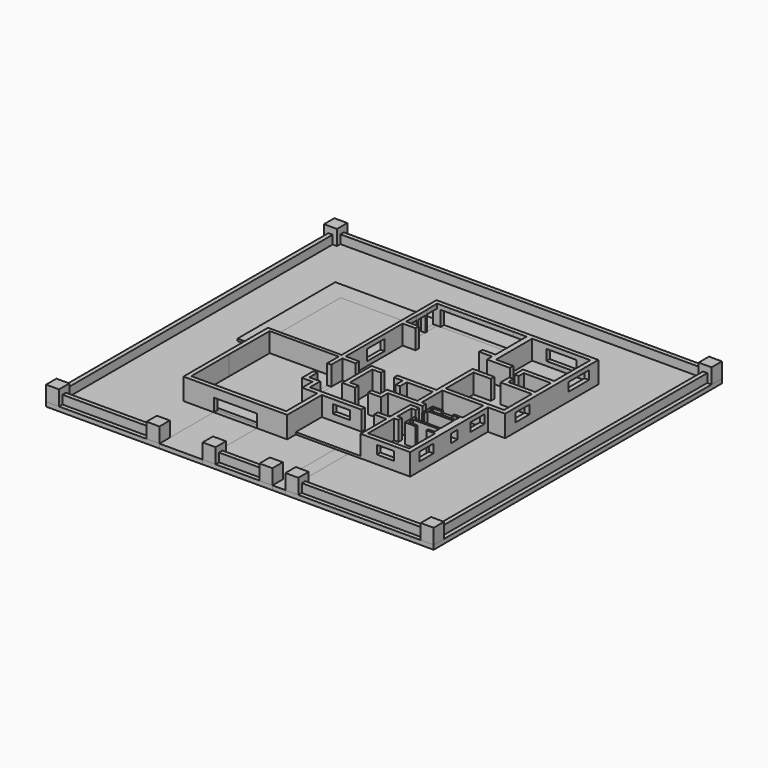
from build123d import *

# Parameters (mm, degrees)
F1_DEPTH  = 254
F2_DEPTH  = 254
F4_DEPTH  = 25.4
F5_W      = 203.2
F5_H      = 177.8
F6_DEPTH  = 50.8
F7_W      = 152.4
F7_H      = 254
F8_DEPTH  = 76.2
F9_W      = 939.5937236786
F9_H      = 25.4
F10_DEPTH = 53.34
F12_DEPTH = 63.5
F14_DEPTH = 76.2
F16_DEPTH = 101.6
F19_DEPTH = 76.2
F21_DEPTH = 76.2
F23_DEPTH = 76.2
F24_W     = 457.2
F24_H     = 177.8
F25_DEPTH = 76.2
F27_DEPTH = 76.2
F28_W     = 25.4
F28_H     = 25.4
F28_H_2   = 50.8
F28_H_3   = 177.8
F29_DEPTH = 50.8
F30_W     = 4055.1800727844
F30_H     = 3734.5069646835
F31_DEPTH = 50.8
F33_W     = 762
F33_H     = 1016
F34_DEPTH = 76.2
F35_W     = 762
F35_H     = 1016
F36_DEPTH = 76.2
F37_W     = 762
F37_H     = 1016
F38_DEPTH = 50.8
F39_DEPTH = 25.4
F40_DEPTH = 508
F41_DEPTH = 254
F42_DEPTH = 254
F44_W     = 3.137548542
F44_H     = 25.4
F44_W_2   = 758.862451458
F45_DEPTH = 381
F46_W     = 152.4
F46_H     = 50.8
F47_DEPTH = 1016
F48_DEPTH = 1016
F49_W     = 152.4
F49_H     = 152.4
F50_DEPTH = 177.8
F52_DEPTH = 1524
F53_W     = 152.4
F53_H     = 152.4
F54_DEPTH = 177.8
F55_W     = 152.4
F55_H     = 152.4
F56_DEPTH = 177.8
F58_DEPTH = 3937
F60_DEPTH = 4318
F62_DEPTH = 4064
F65_DEPTH = 1905
F66_DEPTH = 1905
F67_DEPTH = 799.465
F68_W     = 508
F68_H     = 152.4
F69_DEPTH = 76.2
F70_W     = 152.4
F70_H     = 152.4
F71_DEPTH = 177.8
F72_DEPTH = 1143
F74_DEPTH = 635


with BuildPart() as f1:
    # F0 (on Top) → F1 (new body)
    with BuildSketch(Plane.XY):
        Polygon((177.8, 1192.7142027378), (-304.8, 1192.7142027378), (-635, 1192.7142027378), (-635, 508), (-635, -51.8857972622), (-47.8687277794, -51.8857972622), (587.1312722206, -51.8857972622), (587.1312722206, 456.1142027378), (1349.1312722206, 456.1142027378), (1349.1312722206, 75.1142027378), (1933.3312722206, 75.1142027378), (1933.3312722206, 1218.1142027378), (2136.5312722206, 1218.1142027378), (2136.5312722206, 2589.7142027378), (1349.1312722206, 2589.7142027378), (1179.474234581, 2589.7142027378), (431.8, 2589.7142027378), (231.5312722206, 2589.7142027378), (231.5312722206, 2081.7142027378), (231.5312722206, 1192.7142027378), align=None)
        Polygon((533.4, 0), (0, 0), (-584.2, 0), (-584.2, 558.8), (-581.2687277794, 1150.6002895355), (-301.8687277794, 1150.6002895355), (231.5312722206, 1150.6002895355), (231.5312722206, 608.5142027378), (355.6, 608.5142027378), (355.6, 456.1142027378), (482.6, 456.1142027378), (533.4, 456.1142027378), align=None, mode=Mode.SUBTRACT)
        Polygon((1396.7937236786, 127), (1396.7937236786, 508), (1447.5937236786, 508), (1447.5937236786, 558.8), (1396.7937236786, 558.8), (1396.7937236786, 762), (1447.5937236786, 762), (1447.5937236786, 812.8), (1396.7937236786, 812.8), (1345.9937236786, 812.8), (1345.9937236786, 762), (1345.9937236786, 508), (1041.1937236786, 508), (533.4, 508), (406.4, 508), (406.4, 660.4), (279.4, 660.4), (279.4, 1143), (437.7339612484, 1143), (437.7339612484, 1193.8), (279.4, 1193.8), (279.4, 2032), (431.8, 2032), (431.8, 2081.7142027378), (279.4, 2081.7142027378), (279.4, 2538.9142027378), (431.8, 2538.9142027378), (1179.474234581, 2540), (1331.874234581, 2540), (1331.874234581, 2081.7142027378), (1179.474234581, 2081.7142027378), (1179.474234581, 2032), (1331.874234581, 2032), (1331.874234581, 1957.4247688293), (1600.2, 1957.4247688293), (1600.2, 2008.2247688293), (1396.7937236786, 2008.2247688293), (1396.7937236786, 2540), (2082.5937236786, 2540), (2082.5937236786, 2008.2247688293), (1714.5, 2008.2247688293), (1714.5, 1957.4247688293), (1714.5, 1881.2247688293), (1765.3, 1881.2247688293), (1765.3, 1957.4247688293), (2082.5937236786, 1957.4247688293), (2082.5937236786, 1728.8247688293), (1765.3, 1728.8247688293), (1765.3, 1805.0247688293), (1714.5, 1805.0247688293), (1714.5, 1728.8247688293), (1714.5, 1678.0247688293), (2082.5937236786, 1678.0247688293), (2082.5937236786, 1270), (1828.5937236786, 1270), (1396.7937236786, 1270), (1396.7937236786, 1678.0247688293), (1600.2, 1678.0247688293), (1600.2, 1728.8247688293), (1345.9937236786, 1728.8247688293), (1345.9937236786, 1574.8), (1345.9937236786, 1320.8), (1345.9937236786, 1270), (1345.9937236786, 1193.8), (1193.5937236786, 1193.8), (1039.9870965004, 1193.8), (887.5870965004, 1193.8), (887.5870965004, 1143), (989.1870965004, 1143), (989.1870965004, 1041.4), (1039.9870965004, 1041.4), (1039.9870965004, 1143), (1193.5937236786, 1143), (1345.9937236786, 1143), (1345.9937236786, 1117.6073976807), (1345.9937236786, 939.8), (1345.9937236786, 914.4), (1039.9870965004, 914.4), (989.1870965004, 914.4), (989.1870965004, 812.8), (938.3870965004, 812.8), (887.5870965004, 812.8), (887.5870965004, 762), (1039.9870965004, 762), (1039.9870965004, 812.8), (1039.9870965004, 863.6), (1345.9937236786, 863.6), (1396.7937236786, 863.6), (1447.5937236786, 863.6), (1447.5937236786, 914.4), (1396.7937236786, 914.4), (1396.7937236786, 965.2), (1396.7937236786, 1219.2), (1828.5937236786, 1219.2), (1879.3937236786, 1219.2), (1879.3937236786, 914.4), (1879.3937236786, 811.3352970581), (1879.3937236786, 749.310195446), (1879.3937236786, 508), (1879.3937236786, 127), align=None, mode=Mode.SUBTRACT)
        Polygon((1777.7937236786, 508), (1879.3937236786, 508), (1879.3937236786, 749.310195446), (1879.3937236786, 811.3352970581), (1879.3937236786, 914.4), (1777.7937236786, 914.4), (1777.7937236786, 889), (1853.9937236786, 889), (1853.9937236786, 838.2), (1549.1937236786, 838.2), (1549.1937236786, 889), (1650.7937236786, 889), (1650.7937236786, 914.4), (1523.7937236786, 914.4), (1523.7937236786, 863.6), (1523.7937236786, 811.3352970581), (1523.7937236786, 757.4872970581), (1549.1937236786, 757.4872970581), (1549.1937236786, 811.3352970581), (1853.9937236786, 811.3352970581), (1853.9937236786, 622.3084970581), (1549.1937236786, 622.3084970581), (1549.1937236786, 650.748), (1523.7937236786, 650.748), (1523.7937236786, 596.9), (1523.7937236786, 508), (1650.7937236786, 508), (1650.7937236786, 533.4), (1549.1937236786, 533.4), (1549.1937236786, 596.9), (1853.9937236786, 596.9), (1853.9937236786, 533.4), (1777.7937236786, 533.4), align=None)
    extrude(amount=F1_DEPTH)

    # F0 (on Top) → F2 (join)
    with BuildSketch(Plane.XY):
        Polygon((177.8, 1192.7142027378), (-304.8, 1192.7142027378), (-635, 1192.7142027378), (-635, 508), (-635, -51.8857972622), (-47.8687277794, -51.8857972622), (587.1312722206, -51.8857972622), (587.1312722206, 456.1142027378), (1349.1312722206, 456.1142027378), (1349.1312722206, 75.1142027378), (1933.3312722206, 75.1142027378), (1933.3312722206, 1218.1142027378), (2136.5312722206, 1218.1142027378), (2136.5312722206, 2589.7142027378), (1349.1312722206, 2589.7142027378), (1179.474234581, 2589.7142027378), (431.8, 2589.7142027378), (231.5312722206, 2589.7142027378), (231.5312722206, 2081.7142027378), (231.5312722206, 1192.7142027378), align=None)
        Polygon((533.4, 0), (0, 0), (-584.2, 0), (-584.2, 558.8), (-581.2687277794, 1150.6002895355), (-301.8687277794, 1150.6002895355), (231.5312722206, 1150.6002895355), (231.5312722206, 608.5142027378), (355.6, 608.5142027378), (355.6, 456.1142027378), (482.6, 456.1142027378), (533.4, 456.1142027378), align=None, mode=Mode.SUBTRACT)
        Polygon((1396.7937236786, 127), (1396.7937236786, 508), (1447.5937236786, 508), (1447.5937236786, 558.8), (1396.7937236786, 558.8), (1396.7937236786, 762), (1447.5937236786, 762), (1447.5937236786, 812.8), (1396.7937236786, 812.8), (1345.9937236786, 812.8), (1345.9937236786, 762), (1345.9937236786, 508), (1041.1937236786, 508), (533.4, 508), (406.4, 508), (406.4, 660.4), (279.4, 660.4), (279.4, 1143), (437.7339612484, 1143), (437.7339612484, 1193.8), (279.4, 1193.8), (279.4, 2032), (431.8, 2032), (431.8, 2081.7142027378), (279.4, 2081.7142027378), (279.4, 2538.9142027378), (431.8, 2538.9142027378), (1179.474234581, 2540), (1331.874234581, 2540), (1331.874234581, 2081.7142027378), (1179.474234581, 2081.7142027378), (1179.474234581, 2032), (1331.874234581, 2032), (1331.874234581, 1957.4247688293), (1600.2, 1957.4247688293), (1600.2, 2008.2247688293), (1396.7937236786, 2008.2247688293), (1396.7937236786, 2540), (2082.5937236786, 2540), (2082.5937236786, 2008.2247688293), (1714.5, 2008.2247688293), (1714.5, 1957.4247688293), (1714.5, 1881.2247688293), (1765.3, 1881.2247688293), (1765.3, 1957.4247688293), (2082.5937236786, 1957.4247688293), (2082.5937236786, 1728.8247688293), (1765.3, 1728.8247688293), (1765.3, 1805.0247688293), (1714.5, 1805.0247688293), (1714.5, 1728.8247688293), (1714.5, 1678.0247688293), (2082.5937236786, 1678.0247688293), (2082.5937236786, 1270), (1828.5937236786, 1270), (1396.7937236786, 1270), (1396.7937236786, 1678.0247688293), (1600.2, 1678.0247688293), (1600.2, 1728.8247688293), (1345.9937236786, 1728.8247688293), (1345.9937236786, 1574.8), (1345.9937236786, 1320.8), (1345.9937236786, 1270), (1345.9937236786, 1193.8), (1193.5937236786, 1193.8), (1039.9870965004, 1193.8), (887.5870965004, 1193.8), (887.5870965004, 1143), (989.1870965004, 1143), (989.1870965004, 1041.4), (1039.9870965004, 1041.4), (1039.9870965004, 1143), (1193.5937236786, 1143), (1345.9937236786, 1143), (1345.9937236786, 1117.6073976807), (1345.9937236786, 939.8), (1345.9937236786, 914.4), (1039.9870965004, 914.4), (989.1870965004, 914.4), (989.1870965004, 812.8), (938.3870965004, 812.8), (887.5870965004, 812.8), (887.5870965004, 762), (1039.9870965004, 762), (1039.9870965004, 812.8), (1039.9870965004, 863.6), (1345.9937236786, 863.6), (1396.7937236786, 863.6), (1447.5937236786, 863.6), (1447.5937236786, 914.4), (1396.7937236786, 914.4), (1396.7937236786, 965.2), (1396.7937236786, 1219.2), (1828.5937236786, 1219.2), (1879.3937236786, 1219.2), (1879.3937236786, 914.4), (1879.3937236786, 811.3352970581), (1879.3937236786, 749.310195446), (1879.3937236786, 508), (1879.3937236786, 127), align=None, mode=Mode.SUBTRACT)
    extrude(amount=F2_DEPTH)

    # F5 (on face) → F6 (cut)
    with BuildSketch(Plane(origin=(231.5312722206, 0, 0), x_dir=(0, -1, 0), z_dir=(-1, 0, 0))):
        Polygon((-777.9572461367, 203.2), (-777.9572461367, 254), (-879.5572461367, 254), (-981.1572461367, 254), (-981.1572461367, 203.2), align=None)
        with Locations((-879.5572461367, 114.3)):
            Rectangle(F5_W, F5_H)
    extrude(amount=-F6_DEPTH, mode=Mode.SUBTRACT)

    # F7 (on face) → F8 (cut)
    with BuildSketch(Plane.XZ.offset(-456.1142027378)):
        with Locations((1128.791085434, 127)):
            Rectangle(F7_W, F7_H)
    extrude(amount=-F8_DEPTH, mode=Mode.SUBTRACT)

    # F11 (on face) → F12 (cut)
    with BuildSketch(Plane.XZ.offset(-456.1142027378)):
        Polygon((921.4611788273, 203.2), (819.8611788273, 203.2), (718.2611788273, 203.2), (718.2611788273, 101.6), (921.4611788273, 101.6), align=None)
    extrude(amount=-F12_DEPTH, mode=Mode.SUBTRACT)

    # F13 (on face) → F14 (cut)
    with BuildSketch(Plane.XZ.offset(-75.1142027378)):
        Polygon((1742.8312722206, 203.2), (1641.2312722206, 203.2), (1539.6312722206, 203.2), (1539.6312722206, 101.6), (1742.8312722206, 101.6), align=None)
    extrude(amount=-F14_DEPTH, mode=Mode.SUBTRACT)

    # F15 (on face) → F16 (cut)
    with BuildSketch(Plane.YZ.offset(1933.3312722206)):
        Polygon((418.0142027378, 203.2), (316.4142027378, 203.2), (214.8142027378, 203.2), (214.8142027378, 101.6), (418.0142027378, 101.6), align=None)
        Polygon((1167.3142027378, 203.2), (1065.7142027378, 203.2), (964.1142027378, 203.2), (964.1142027378, 101.6), (1167.3142027378, 101.6), align=None)
        Polygon((773.6142027378, 203.2), (710.1142027378, 203.2), (672.0142027378, 203.2), (672.0142027378, 101.6), (773.6142027378, 101.6), align=None)
    extrude(amount=-F16_DEPTH, mode=Mode.SUBTRACT)

    # F18 (on face) → F19 (cut)
    with BuildSketch(Plane.YZ.offset(2136.5312722206)):
        Polygon((2452.1544022799, 203.2), (2299.7544022799, 203.2), (2147.3544022799, 203.2), (2147.3544022799, 101.6), (2452.1544022799, 101.6), align=None)
        Polygon((1573.7142027378, 203.2), (1472.1142027378, 203.2), (1370.5142027378, 203.2), (1370.5142027378, 101.6), (1573.7142027378, 101.6), align=None)
    extrude(amount=-F19_DEPTH, mode=Mode.SUBTRACT)

    # F20 (on face) → F21 (cut)
    with BuildSketch(Plane(origin=(0, 2589.7142027378, 0), x_dir=(-1, 0, 0), z_dir=(0, 1, 0))):
        Polygon((-1565.0312722206, 203.2), (-1742.8312722206, 203.2), (-1920.6312722206, 203.2), (-1920.6312722206, 76.2), (-1565.0312722206, 76.2), align=None)
    extrude(amount=-F21_DEPTH, mode=Mode.SUBTRACT)

    # F22 (on face) → F23 (cut)
    with BuildSketch(Plane(origin=(0, 2589.7142027378, 0), x_dir=(-1, 0, 0), z_dir=(0, 1, 0))):
        Polygon((-320.4312722206, 203.2), (-803.0312722206, 203.2), (-1285.6312722206, 203.2), (-1285.6312722206, 25.4), (-320.4312722206, 25.4), align=None)
    extrude(amount=-F23_DEPTH, mode=Mode.SUBTRACT)

    # F24 (on face) → F25 (cut)
    with BuildSketch(Plane(origin=(231.5312722206, 0, 0), x_dir=(0, -1, 0), z_dir=(-1, 0, 0))):
        with Locations((-2310.3142027378, 114.3)):
            Rectangle(F24_W, F24_H)
    extrude(amount=-F25_DEPTH, mode=Mode.SUBTRACT)

    # F26 (on face) → F27 (cut)
    with BuildSketch(Plane(origin=(231.5312722206, 0, 0), x_dir=(0, -1, 0), z_dir=(-1, 0, 0))):
        Polygon((-1510.2142027378, 203.2), (-1764.2142027378, 203.2), (-1764.2142027378, 76.2), (-1637.2142027378, 76.2), (-1510.2142027378, 76.2), align=None)
    extrude(amount=-F27_DEPTH, mode=Mode.SUBTRACT)



with BuildPart() as f2:
    # F0 (on Top) → F2, piece 2 (new body)
    with BuildSketch(Plane.XY):
        Polygon((582.7870965004, 762), (735.1870965004, 762), (735.1870965004, 812.8), (633.5870965004, 812.8), (633.5870965004, 1143), (735.1870965004, 1143), (735.1870965004, 1193.8), (582.7870965004, 1193.8), (582.7870965004, 1143), (582.7870965004, 812.8), align=None)
    extrude(amount=F2_DEPTH)


with BuildPart() as f4:
    # F3 (on face) → F4 (new body)
    with BuildSketch(Plane(origin=(0, 0, 0), x_dir=(1, 0, 0), z_dir=(0, 0, -1))):
        Polygon((533.4, -456.1142027378), (533.4, 0), (-584.2, 0), (-584.2, -558.8), (-581.2687277794, -1150.6002895355), (231.5312722206, -1150.6002895355), (231.5312722206, -608.5142027378), (355.6, -608.5142027378), (355.6, -456.1142027378), align=None)
    extrude(amount=-F4_DEPTH)


with BuildPart() as f4b:
    # F3 (on face) → F4, piece 2 (new body)
    with BuildSketch(Plane(origin=(0, 0, 0), x_dir=(1, 0, 0), z_dir=(0, 0, -1))):
        Polygon((1039.9870965004, -762), (1039.9870965004, -863.6), (1447.5937236786, -863.6), (1447.5937236786, -914.4), (1396.7937236786, -914.4), (1396.7937236786, -1219.2), (1879.3937236786, -1219.2), (1879.3937236786, -914.4), (1777.7937236786, -914.4), (1777.7937236786, -889), (1853.9937236786, -889), (1853.9937236786, -838.2), (1549.1937236786, -838.2), (1549.1937236786, -889), (1650.7937236786, -889), (1650.7937236786, -914.4), (1523.7937236786, -914.4), (1523.7937236786, -757.4872970581), (1549.1937236786, -757.4872970581), (1549.1937236786, -811.3352970581), (1853.9937236786, -811.3352970581), (1853.9937236786, -622.3084970581), (1549.1937236786, -622.3084970581), (1549.1937236786, -650.748), (1523.7937236786, -650.748), (1523.7937236786, -508), (1650.7937236786, -508), (1650.7937236786, -533.4), (1549.1937236786, -533.4), (1549.1937236786, -596.9), (1853.9937236786, -596.9), (1853.9937236786, -533.4), (1777.7937236786, -533.4), (1777.7937236786, -508), (1879.3937236786, -508), (1879.3937236786, -127), (1396.7937236786, -127), (1396.7937236786, -508), (1447.5937236786, -508), (1447.5937236786, -558.8), (1396.7937236786, -558.8), (1396.7937236786, -762), (1447.5937236786, -762), (1447.5937236786, -812.8), (1345.9937236786, -812.8), (1345.9937236786, -508), (406.4, -508), (406.4, -660.4), (279.4, -660.4), (279.4, -1143), (437.7339612484, -1143), (437.7339612484, -1193.8), (279.4, -1193.8), (279.4, -2032), (431.8, -2032), (431.8, -2081.7142027378), (279.4, -2081.7142027378), (279.4, -2538.9142027378), (431.8, -2538.9142027378), (1179.474234581, -2540), (1331.874234581, -2540), (1331.874234581, -2081.7142027378), (1179.474234581, -2081.7142027378), (1179.474234581, -2032), (1331.874234581, -2032), (1331.874234581, -1957.4247688293), (1600.2, -1957.4247688293), (1600.2, -2008.2247688293), (1396.7937236786, -2008.2247688293), (1396.7937236786, -2540), (2082.5937236786, -2540), (2082.5937236786, -2008.2247688293), (1714.5, -2008.2247688293), (1714.5, -1881.2247688293), (1765.3, -1881.2247688293), (1765.3, -1957.4247688293), (2082.5937236786, -1957.4247688293), (2082.5937236786, -1728.8247688293), (1765.3, -1728.8247688293), (1765.3, -1805.0247688293), (1714.5, -1805.0247688293), (1714.5, -1678.0247688293), (2082.5937236786, -1678.0247688293), (2082.5937236786, -1270), (1396.7937236786, -1270), (1396.7937236786, -1678.0247688293), (1600.2, -1678.0247688293), (1600.2, -1728.8247688293), (1345.9937236786, -1728.8247688293), (1345.9937236786, -1193.8), (887.5870965004, -1193.8), (887.5870965004, -1143), (989.1870965004, -1143), (989.1870965004, -1041.4), (1039.9870965004, -1041.4), (1039.9870965004, -1143), (1345.9937236786, -1143), (1345.9937236786, -914.4), (989.1870965004, -914.4), (989.1870965004, -812.8), (887.5870965004, -812.8), (887.5870965004, -762), align=None)
    extrude(amount=-F4_DEPTH)


with BuildPart() as f10:
    # F9 (on face) → F10 (new body)
    with BuildSketch(Plane.XZ.offset(-508)):
        with Locations((876.1968618393, 12.7)):
            Rectangle(F9_W, F9_H)
    extrude(amount=F10_DEPTH)


with BuildPart() as f29:
    # F28 (on face) → F29 (new body)
    with BuildSketch(Plane(origin=(231.5312722206, 0, 0), x_dir=(0, -1, 0), z_dir=(-1, 0, 0))):
        with Locations((-2246.8142027378, 12.7)):
            Rectangle(F28_W, F28_H)
        with Locations((-2246.8142027378, 228.6)):
            Rectangle(F28_W, F28_H_2)
        with Locations((-2246.8142027378, 114.3)):
            Rectangle(F28_W, F28_H_3)
        Polygon((-2361.1142027378, 254), (-2361.1142027378, 203.2), (-2310.3142027378, 203.2), (-2259.5142027378, 203.2), (-2259.5142027378, 254), align=None)
        with Locations((-2373.8142027378, 114.3)):
            Rectangle(F28_W, F28_H_3)
        with Locations((-2373.8142027378, 228.6)):
            Rectangle(F28_W, F28_H_2)
        Polygon((-2310.3142027378, 25.4), (-2361.1142027378, 25.4), (-2386.5142027378, 25.4), (-2386.5142027378, 0), (-2259.5142027378, 0), (-2259.5142027378, 25.4), align=None)
    extrude(amount=-F29_DEPTH)


with BuildPart() as f31:
    # F30 (on face) → F31 (new body)
    with BuildSketch(Plane(origin=(0, 0, 0), x_dir=(1, 0, 0), z_dir=(0, 0, -1))):
        with Locations((922.8382110596, -1270.1082825661)):
            Rectangle(F30_W, F30_H)
        Polygon((2136.5312722206, -2589.7142027378), (231.5312722206, -2589.7142027378), (231.5312722206, -1192.7142027378), (-635, -1192.7142027378), (-635, 51.8857972622), (587.1312722206, 51.8857972622), (587.1312722206, -456.1142027378), (1052.591085434, -456.1142027378), (1052.591085434, -508), (406.4, -508), (406.4, -660.4), (279.4, -660.4), (279.4, -1143), (437.7339612484, -1143), (437.7339612484, -1193.8), (279.4, -1193.8), (279.4, -2032), (431.8, -2032), (431.8, -2081.7142027378), (279.4, -2081.7142027378), (279.4, -2538.9142027378), (431.8, -2538.9142027378), (1179.474234581, -2540), (1331.874234581, -2540), (1331.874234581, -2081.7142027378), (1179.474234581, -2081.7142027378), (1179.474234581, -2032), (1331.874234581, -2032), (1331.874234581, -1957.4247688293), (1600.2, -1957.4247688293), (1600.2, -2008.2247688293), (1396.7937236786, -2008.2247688293), (1396.7937236786, -2540), (2082.5937236786, -2540), (2082.5937236786, -2008.2247688293), (1714.5, -2008.2247688293), (1714.5, -1881.2247688293), (1765.3, -1881.2247688293), (1765.3, -1957.4247688293), (2082.5937236786, -1957.4247688293), (2082.5937236786, -1728.8247688293), (1765.3, -1728.8247688293), (1765.3, -1805.0247688293), (1714.5, -1805.0247688293), (1714.5, -1678.0247688293), (2082.5937236786, -1678.0247688293), (2082.5937236786, -1270), (1396.7937236786, -1270), (1396.7937236786, -1678.0247688293), (1600.2, -1678.0247688293), (1600.2, -1728.8247688293), (1345.9937236786, -1728.8247688293), (1345.9937236786, -1193.8), (887.5870965004, -1193.8), (887.5870965004, -1143), (989.1870965004, -1143), (989.1870965004, -1041.4), (1039.9870965004, -1041.4), (1039.9870965004, -1143), (1345.9937236786, -1143), (1345.9937236786, -914.4), (989.1870965004, -914.4), (989.1870965004, -812.8), (887.5870965004, -812.8), (887.5870965004, -762), (1039.9870965004, -762), (1039.9870965004, -863.6), (1447.5937236786, -863.6), (1447.5937236786, -914.4), (1396.7937236786, -914.4), (1396.7937236786, -1219.2), (1879.3937236786, -1219.2), (1879.3937236786, -914.4), (1777.7937236786, -914.4), (1777.7937236786, -889), (1853.9937236786, -889), (1853.9937236786, -838.2), (1549.1937236786, -838.2), (1549.1937236786, -889), (1650.7937236786, -889), (1650.7937236786, -914.4), (1523.7937236786, -914.4), (1523.7937236786, -757.4872970581), (1549.1937236786, -757.4872970581), (1549.1937236786, -811.3352970581), (1853.9937236786, -811.3352970581), (1853.9937236786, -622.3084970581), (1549.1937236786, -622.3084970581), (1549.1937236786, -650.748), (1523.7937236786, -650.748), (1523.7937236786, -508), (1650.7937236786, -508), (1650.7937236786, -533.4), (1549.1937236786, -533.4), (1549.1937236786, -596.9), (1853.9937236786, -596.9), (1853.9937236786, -533.4), (1777.7937236786, -533.4), (1777.7937236786, -508), (1879.3937236786, -508), (1879.3937236786, -127), (1396.7937236786, -127), (1396.7937236786, -508), (1447.5937236786, -508), (1447.5937236786, -558.8), (1396.7937236786, -558.8), (1396.7937236786, -762), (1447.5937236786, -762), (1447.5937236786, -812.8), (1345.9937236786, -812.8), (1345.9937236786, -508), (1204.991085434, -508), (1204.991085434, -456.1142027378), (1349.1312722206, -456.1142027378), (1349.1312722206, -75.1142027378), (1933.3312722206, -75.1142027378), (1933.3312722206, -1218.1142027378), (2136.5312722206, -1218.1142027378), align=None, mode=Mode.SUBTRACT)
    extrude(amount=F31_DEPTH)

    # F33 (on face) → F34 (cut)
    with BuildSketch(Plane.XY):
        with Locations((-381, 1911.4676551819)):
            Rectangle(F33_W, F33_H)
    extrude(amount=-F34_DEPTH, mode=Mode.SUBTRACT)

    # F40 (add): a face of the model
    f40_faces = [f31.faces().sort_by_distance(p)[0] for p in [
        (-1104.7518253326, 1270.1082825661, -25.4),
    ]]
    extrude(f40_faces, amount=F40_DEPTH)

    # F41 (add): a face of the model
    f41_faces = [f31.faces().sort_by_distance(p)[0] for p in [
        (668.8382110596, -597.1451997757, -25.4),
    ]]
    extrude(f41_faces, amount=F41_DEPTH)

    # F42 (add): a face of the model
    f42_faces = [f31.faces().sort_by_distance(p)[0] for p in [
        (668.8382110596, 3137.3617649078, -25.4),
    ]]
    extrude(f42_faces, amount=F42_DEPTH)

    # F46 (on face) → F47 (cut)
    with BuildSketch(Plane.XZ.offset(851.1451997757)):
        with Locations((1128.791085434, -25.4)):
            Rectangle(F46_W, F46_H)
    extrude(amount=-F47_DEPTH, mode=Mode.SUBTRACT)


with BuildPart() as f31b:
    # F30 (on face) → F31, piece 2 (new body)
    with BuildSketch(Plane(origin=(0, 0, 0), x_dir=(1, 0, 0), z_dir=(0, 0, -1))):
        Polygon((533.4, -456.1142027378), (533.4, 0), (-584.2, 0), (-584.2, -558.8), (-581.2687277794, -1150.6002895355), (231.5312722206, -1150.6002895355), (231.5312722206, -608.5142027378), (355.6, -608.5142027378), (355.6, -456.1142027378), align=None)
    extrude(amount=F31_DEPTH)


with BuildPart() as f36:
    # F35 (on face) → F36 (new body)
    with BuildSketch(Plane(origin=(0, 0, -50.8), x_dir=(1, 0, 0), z_dir=(0, 0, -1))):
        with Locations((-381, -1911.4676551819)):
            Rectangle(F35_W, F35_H)
    extrude(amount=-F36_DEPTH)


with BuildPart() as f38:
    # F37 (on face) → F38 (new body)
    with BuildSketch(Plane.XY):
        Polygon((231.5312722206, 1192.7142027378), (231.5312722206, 2589.7142027378), (231.5312722206, 2630.2114551819), (-993.521, 2630.2114551819), (-993.521, 2419.4676551819), (-993.521, 1192.7142027378), (-762, 1192.7142027378), (-635, 1192.7142027378), align=None)
        with Locations((-381, 1911.4676551819)):
            Rectangle(F37_W, F37_H, mode=Mode.SUBTRACT)
    extrude(amount=-F38_DEPTH)


with BuildPart() as f39:
    # F39 (new): a face of the model
    f39_faces = [f38.part.faces().sort_by_distance(p)[0] for p in [
        (212.6443682381, 1911.4628289598, 0),
    ]]
    extrude(f39_faces, amount=F39_DEPTH)


with BuildPart() as f45:
    # F44 (on face) → F45 (new body)
    with BuildSketch(Plane.XZ.offset(-454.66)):
        with Locations((1347.5624979496, 12.7)):
            Rectangle(F44_W, F44_H)
        with Locations((966.5624979496, 12.7)):
            Rectangle(F44_W_2, F44_H)
    extrude(amount=F45_DEPTH)


with BuildPart() as f48:
    # F48 (new): a face of the model
    f48_faces = [f31.part.faces().sort_by_distance(p)[0] for p in [
        (1128.791085434, 164.8548002243, -25.4),
    ]]
    extrude(f48_faces, amount=F48_DEPTH)


with BuildPart() as f50:
    # F49 (on face) → F50 (new body)
    with BuildSketch(Plane.XY):
        with Locations((976.391085434, -774.9451997757)):
            Rectangle(F49_W, F49_H)
    extrude(amount=F50_DEPTH)


with BuildPart() as f50b:
    # F49 (on face) → F50, piece 2 (new body)
    with BuildSketch(Plane.XY):
        with Locations((1281.191085434, -774.9451997757)):
            Rectangle(F49_W, F49_H)
    extrude(amount=F50_DEPTH)


with BuildPart() as f52:
    # F51 (on face) → F52 (new body)
    with BuildSketch(Plane.YZ.offset(1357.391085434)):
        Polygon((-800.3451997757, 101.6), (-800.3451997757, 0), (-774.9451997757, 0), (-749.5451997757, 0), (-749.5451997757, 101.6), align=None)
    extrude(amount=F52_DEPTH)


with BuildPart() as f54:
    # F53 (on face) → F54 (new body)
    with BuildSketch(Plane.XY):
        with Locations((2874.2282474518, -774.9451997757)):
            Rectangle(F53_W, F53_H)
    extrude(amount=F54_DEPTH)


with BuildPart() as f56:
    # F55 (on face) → F56 (new body)
    with BuildSketch(Plane.XY):
        with Locations((2874.2282474518, 3315.1617649078)):
            Rectangle(F55_W, F55_H)
    extrude(amount=F56_DEPTH)


with BuildPart() as f56b:
    # F55 (on face) → F56, piece 2 (new body)
    with BuildSketch(Plane.XY):
        with Locations((-1536.5518253326, 3315.1617649078)):
            Rectangle(F55_W, F55_H)
    extrude(amount=F56_DEPTH)


with BuildPart() as f56c:
    # F55 (on face) → F56, piece 3 (new body)
    with BuildSketch(Plane.XY):
        with Locations((-1536.5518253326, -774.9451997757)):
            Rectangle(F55_W, F55_H)
    extrude(amount=F56_DEPTH)


with BuildPart() as f58:
    # F57 (on face) → F58 (new body)
    with BuildSketch(Plane.XZ.offset(-3238.9617649078)):
        Polygon((2848.8282474518, 101.6), (2848.8282474518, 0), (2874.2282474518, 0), (2899.6282474518, 0), (2899.6282474518, 101.6), align=None)
    extrude(amount=F58_DEPTH)


with BuildPart() as f60:
    # F59 (on face) → F60 (new body)
    with BuildSketch(Plane.YZ.offset(-1460.3518253326)):
        Polygon((3289.7617649078, 0), (3315.1617649078, 0), (3340.5617649078, 0), (3340.5617649078, 101.6), (3289.7617649078, 101.6), align=None)
    extrude(amount=F60_DEPTH)


with BuildPart() as f62:
    # F61 (on face) → F62 (new body)
    with BuildSketch(Plane.XZ.offset(-3238.9617649078)):
        Polygon((-1561.9518253326, 0), (-1536.5518253326, 0), (-1511.1518253326, 0), (-1511.1518253326, 101.6), (-1561.9518253326, 101.6), align=None)
    extrude(amount=F62_DEPTH)


with BuildPart() as f1_1:
    add(f1.part)

    add(f31.part)  # F65 merges F31
    # F64 (on face) → F65 (join)
    with BuildSketch(Plane.XZ.offset(51.8857972622)):
        Polygon((230.0656361103, 0), (-23.9343638897, 0), (-277.9343638897, 0), (-277.9343638897, -50.8), (230.0656361103, -50.8), align=None)
    extrude(amount=F65_DEPTH)

    # F66 (cut): a face of the model
    f66_faces = [f1_1.faces().sort_by_distance(p)[0] for p in [
        (-23.9343638897, -1956.8857972622, -25.4),
    ]]
    extrude(f66_faces, amount=-F66_DEPTH, mode=Mode.SUBTRACT)

    # F68 (on face) → F69 (cut)
    with BuildSketch(Plane.XZ.offset(51.8857972622)):
        with Locations((-23.9343638897, 76.2)):
            Rectangle(F68_W, F68_H)
    extrude(amount=-F69_DEPTH, mode=Mode.SUBTRACT)


with BuildPart() as f67:
    # F64 (on face) → F67 (new body)
    with BuildSketch(Plane.XZ.offset(51.8857972622)):
        Polygon((230.0656361103, 0), (-23.9343638897, 0), (-277.9343638897, 0), (-277.9343638897, -50.8), (230.0656361103, -50.8), align=None)
    extrude(amount=F67_DEPTH)


with BuildPart() as f71:
    # F70 (on face) → F71 (new body)
    with BuildSketch(Plane.XY):
        with Locations((-354.1343638897, -774.9451997757)):
            Rectangle(F70_W, F70_H)
    extrude(amount=F71_DEPTH)


with BuildPart() as f71b:
    # F70 (on face) → F71, piece 2 (new body)
    with BuildSketch(Plane.XY):
        with Locations((306.2656361103, -774.9451997757)):
            Rectangle(F70_W, F70_H)
    extrude(amount=F71_DEPTH)


with BuildPart() as f72:
    # F63 (on face) → F72 (new body)
    with BuildSketch(Plane.YZ.offset(-1460.3518253326)):
        Polygon((-800.3451997757, 0), (-774.9451997757, 0), (-749.5451997757, 0), (-749.5451997757, 101.6), (-800.3451997757, 101.6), align=None)
    extrude(amount=F72_DEPTH)


with BuildPart() as f74:
    # F73 (on face) → F74 (new body)
    with BuildSketch(Plane.YZ.offset(382.4656361103)):
        Polygon((-800.3451997757, 0), (-774.9451997757, 0), (-749.5451997757, 0), (-749.5451997757, 101.6), (-800.3451997757, 101.6), align=None)
    extrude(amount=F74_DEPTH)


solid = Compound([f2.part, f4.part, f4b.part, f10.part, f29.part, f31b.part, f36.part, f38.part, f39.part, f45.part, f48.part, f50.part, f50b.part, f52.part, f54.part, f56.part, f56b.part, f56c.part, f58.part, f60.part, f62.part, f1_1.part, f67.part, f71.part, f71b.part, f72.part, f74.part])
